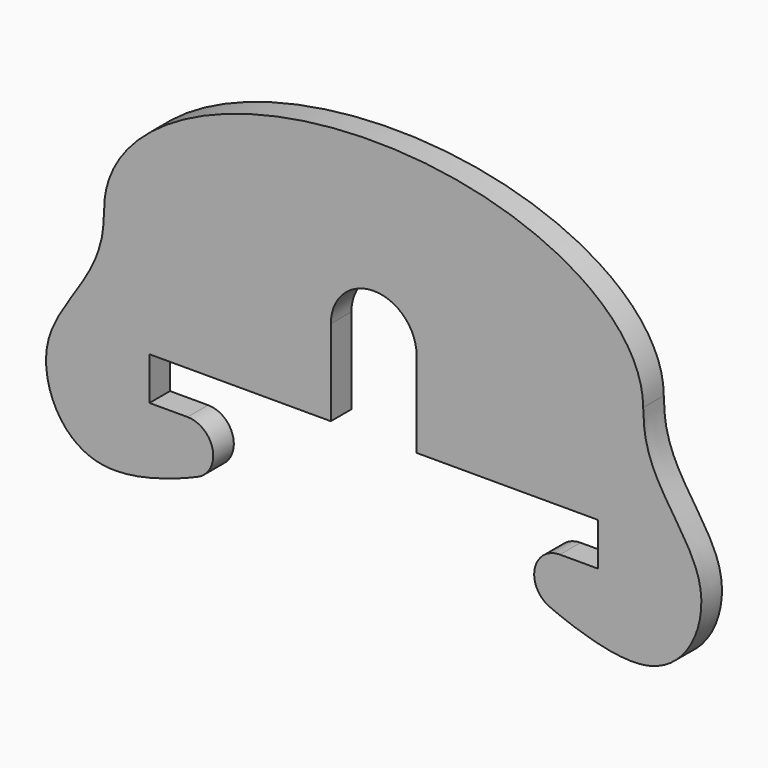
from build123d import *

# Parameters (mm, degrees)
F1_DEPTH = 3


# Not quite as in the source:
# - ends of sketch curves that miss each other by under 0.0002 mm in the source are joined
# - the dataset's text gives a spline's control points without its knots; the knots are read off the source's solid


with BuildPart() as f1:
    # F0 (on Front) → F1 (new body)
    with BuildSketch(Plane.XZ):
        with BuildLine():
            Line((-21.706138, -13.579078), (-26.14, -13.579078))
            Line((-26.14, -13.579078), (-26.14, -8.579078))
            Line((-26.14, -8.579078), (-5, -8.579078))
            Line((-5, -8.579078), (-5, 1.420922))
            ThreePointArc((-5, 1.420922), (0, 6.420922), (5, 1.420922))
            Line((5, 1.420922), (5, -8.579078))
            Line((5, -8.579078), (26.14, -8.579078))
            Line((26.14, -8.579078), (26.14, -13.579078))
            Line((26.14, -13.579078), (21.706137, -13.579078))
            ThreePointArc((21.706137, -13.579078), (18.7680952866, -15.9725214153), (20.5180779685, -19.3338040731))
            add(Edge.make_bspline(
                [(31.409969, 4.662538), (31.457769, 4.179313), (31.482006, -2.918842), (41.55044, -9.601034), (34.658633, -24.650185), (23.26845, -20.519985), (20.5180779685, -19.3338040731)],
                knots=[26.688985, 26.688985, 26.688985, 26.688985, 28.557776, 42.872008, 54.1154, 62.665306, 62.665306, 62.665306, 62.665306], degree=3))
            add(Edge.make_bspline(
                [(31.409969, 4.662538), (31.409969, 21.7909259667), (-5.4404e-06, 21.790923), (-31.4099798807, 21.7909200333), (-31.409969, 4.6625320666)],
                knots=[0, 0, 0, 1.5707965, 1.5707965, 3.141593, 3.141593, 3.141593], degree=2, weights=[1, 0.7071067199, 1, 0.7071067199, 1]))
            add(Edge.make_bspline(
                [(-31.409969, 4.6625320666), (-31.457769, 4.179313), (-31.482006, -2.918842), (-41.55044, -9.601034), (-34.658633, -24.650185), (-23.268451, -20.519985), (-20.518078, -19.333804)],
                knots=[26.688985, 26.688985, 26.688985, 26.688985, 28.557776, 42.872008, 54.1154, 62.665306, 62.665306, 62.665306, 62.665306], degree=3))
            ThreePointArc((-20.518078, -19.333804), (-18.7680963794, -15.9725209657), (-21.706138, -13.579078))
        make_face()
    extrude(amount=F1_DEPTH)


solid = f1.part
